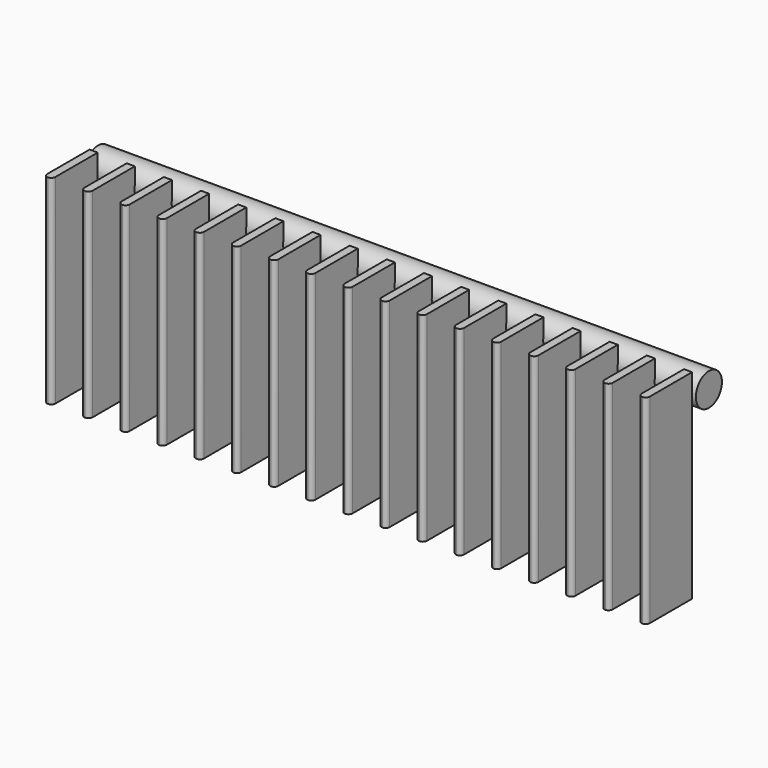
from build123d import *

# Parameters (mm, degrees)
F0_R          = 20
F1_DEPTH      = 375
F3_W          = 10
F3_H          = 70
F4_DEPTH      = 25
F4_DEPTH_BACK = 220
F5_R          = 4.99999
F6_R          = 4.99999


# Not quite as in the source:
# - a fillet or chamfer is up to 0.001 mm smaller than in the source, because OpenCascade refuses the exact size
# - a feature names something its author has since deleted; it is built from what else it names


with BuildPart() as f1:
    # F0 (on Right) → F1 (new body, symmetric)
    with BuildSketch(Plane.YZ):
        with Locations((-45, 220)):
            Circle(F0_R)
    extrude(amount=F1_DEPTH, both=True)

    # F3 (on plane+point) → F4 (join, two sides)
    with BuildSketch(Plane.XY.offset(220)) as f4_sk:
        with Locations((-365, -99.5)):
            Rectangle(F3_W, F3_H)
        with Locations((-319.375, -99.5)):
            Rectangle(F3_W, F3_H)
        with Locations((-273.75, -99.5)):
            Rectangle(F3_W, F3_H)
        with Locations((-228.125, -99.5)):
            Rectangle(F3_W, F3_H)
        with Locations((-182.5, -99.5)):
            Rectangle(F3_W, F3_H)
        with Locations((-136.875, -99.5)):
            Rectangle(F3_W, F3_H)
        with Locations((-91.25, -99.5)):
            Rectangle(F3_W, F3_H)
        with Locations((-45.625, -99.5)):
            Rectangle(F3_W, F3_H)
        with Locations((0, -99.5)):
            Rectangle(F3_W, F3_H)
        with Locations((45.625, -99.5)):
            Rectangle(F3_W, F3_H)
        with Locations((91.25, -99.5)):
            Rectangle(F3_W, F3_H)
        with Locations((136.875, -99.5)):
            Rectangle(F3_W, F3_H)
        with Locations((182.5, -99.5)):
            Rectangle(F3_W, F3_H)
        with Locations((228.125, -99.5)):
            Rectangle(F3_W, F3_H)
        with Locations((273.75, -99.5)):
            Rectangle(F3_W, F3_H)
        with Locations((319.375, -99.5)):
            Rectangle(F3_W, F3_H)
        with Locations((365, -99.5)):
            Rectangle(F3_W, F3_H)
    extrude(amount=F4_DEPTH)
    extrude(f4_sk.sketch, amount=-F4_DEPTH_BACK)

    # F5 (radius 5 in the source; OpenCascade refuses exactly that, so slightly less here)
    f5_edges = [f1.edges().sort_by_distance(p)[0] for p in [
        (-360, -134.5, 122.5),
        (-370, -134.5, 122.5),
    ]]
    fillet(f5_edges, radius=F5_R)

    # F6 (radius 5 in the source; OpenCascade refuses exactly that, so slightly less here)
    f6_edges = [f1.edges().sort_by_distance(p)[0] for p in [
        (-324.375, -134.5, 122.5),
        (-314.375, -134.5, 122.5),
        (-278.75, -134.5, 122.5),
        (-268.75, -134.5, 122.5),
        (-223.125, -134.5, 122.5),
        (-233.125, -134.5, 122.5),
        (-177.5, -134.5, 122.5),
        (-187.5, -134.5, 122.5),
        (-131.875, -134.5, 122.5),
        (-141.875, -134.5, 122.5),
        (-86.25, -134.5, 122.5),
        (-96.25, -134.5, 122.5),
        (-40.625, -134.5, 122.5),
        (-50.625, -134.5, 122.5),
        (5, -134.5, 122.5),
        (-5, -134.5, 122.5),
        (50.625, -134.5, 122.5),
        (40.625, -134.5, 122.5),
        (86.25, -134.5, 122.5),
        (96.25, -134.5, 122.5),
        (131.875, -134.5, 122.5),
        (141.875, -134.5, 122.5),
        (187.5, -134.5, 122.5),
        (177.5, -134.5, 122.5),
        (233.125, -134.5, 122.5),
        (223.125, -134.5, 122.5),
        (278.75, -134.5, 122.5),
        (268.75, -134.5, 122.5),
        (324.375, -134.5, 122.5),
        (314.375, -134.5, 122.5),
        (370, -134.5, 122.5),
        (360, -134.5, 122.5),
    ]]
    fillet(f6_edges, radius=F6_R)


solid = f1.part
